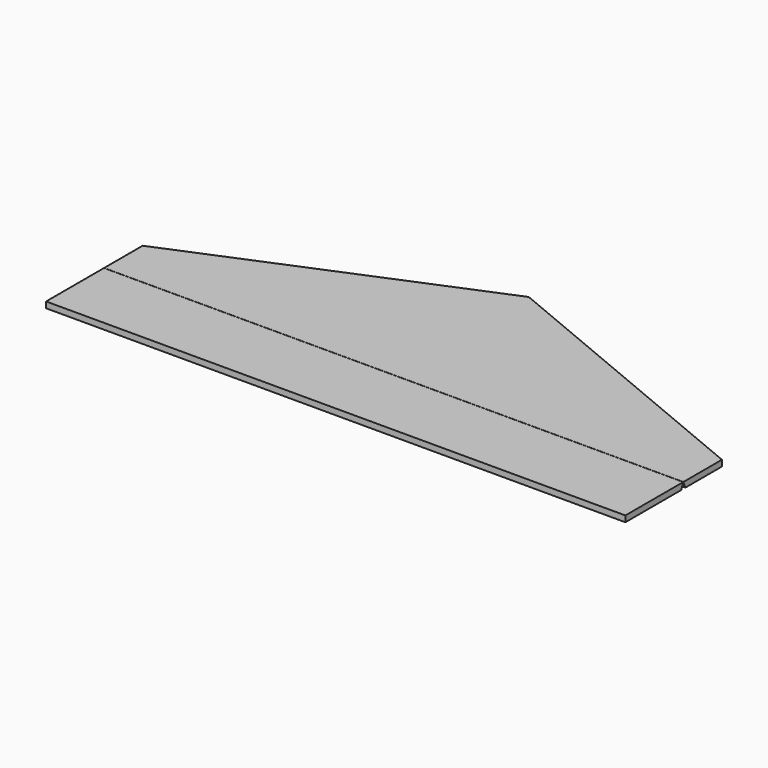
from build123d import *

# Parameters (mm, degrees)
F1_DEPTH    = 3.175
F0_W        = 152.4
F0_H        = 38.1
F2_DEPTH    = 3.175
F3_T1_DEPTH = 321.9219952748
F4_T1_DEPTH = 321.9219952748


# Not quite as in the source:
# - a fillet or chamfer that OpenCascade refuses, or shapes differently, is made with other operations: its cross-section is extruded or revolved along the edge and cut away or added


with BuildPart() as f1:
    # F0 (on Top) → F1 (new body)
    with BuildSketch(Plane.XY):
        Polygon((-152.4, 25.4), (-152.4, 0), (0, 0), (0, 88.9), align=None)
        Polygon((0, 88.9), (0, 0), (152.4, 0), (152.4, 25.4), align=None)
    extrude(amount=F1_DEPTH)

    # F3: chamfer of 3.302 x 1.367733183 on 1 edges, made by hand

    # F3_s2 → F3_t1 (cut)
    with BuildSketch(Plane.YZ.offset(-160.9609976374)):
        Polygon((0, 3.302), (1.367733183, 0), (0, 0), align=None)
    extrude(amount=F3_T1_DEPTH, mode=Mode.SUBTRACT)


with BuildPart() as f2:
    # F0 (on Top) → F2 (new body)
    with BuildSketch(Plane.XY):
        with Locations((-76.2, -19.05)):
            Rectangle(F0_W, F0_H)
        with Locations((76.2, -19.05)):
            Rectangle(F0_W, F0_H)
    extrude(amount=F2_DEPTH)

    # F4: chamfer of 3.302 x 1.367733183 on 1 edges, made by hand

    # F4_s2 → F4_t1 (cut)
    with BuildSketch(Plane.YZ.offset(-160.9609976374)):
        Polygon((0, 3.302), (-1.367733183, 0), (0, 0), align=None)
    extrude(amount=F4_T1_DEPTH, mode=Mode.SUBTRACT)


solid = Compound([f1.part, f2.part])
